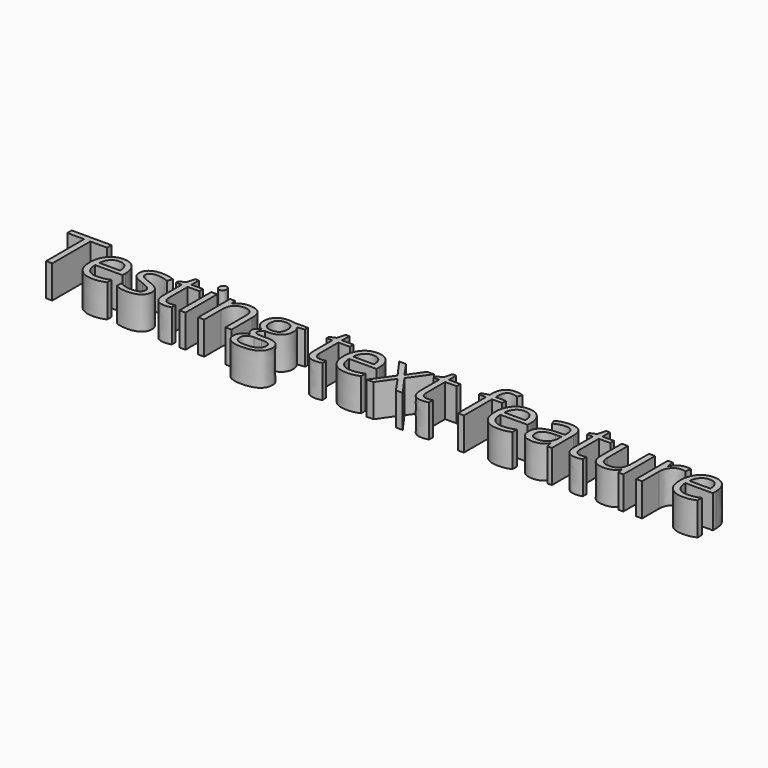
from build123d import *

# Parameters (mm, degrees)
F0_TEXT_SIZE = 57.64320441
F1_DEPTH     = 25.4


# Not quite as in the source:
# - Text() gives the source's letters only with a copy of the font that has no kerning and outlines rounded to 1/6400 em; it was checked with that copy


with BuildPart() as f1:
    # F0 (on Top) → F1 (new body)
    with BuildSketch(Plane.XY):
        with Locations((-223.7172797322, -32.4034933001)):
            Text('Testing text feature', F0_TEXT_SIZE, font='Open Sans', text_align=(TextAlign.LEFT, TextAlign.BOTTOM))
    extrude(amount=F1_DEPTH)


solid = f1.part
